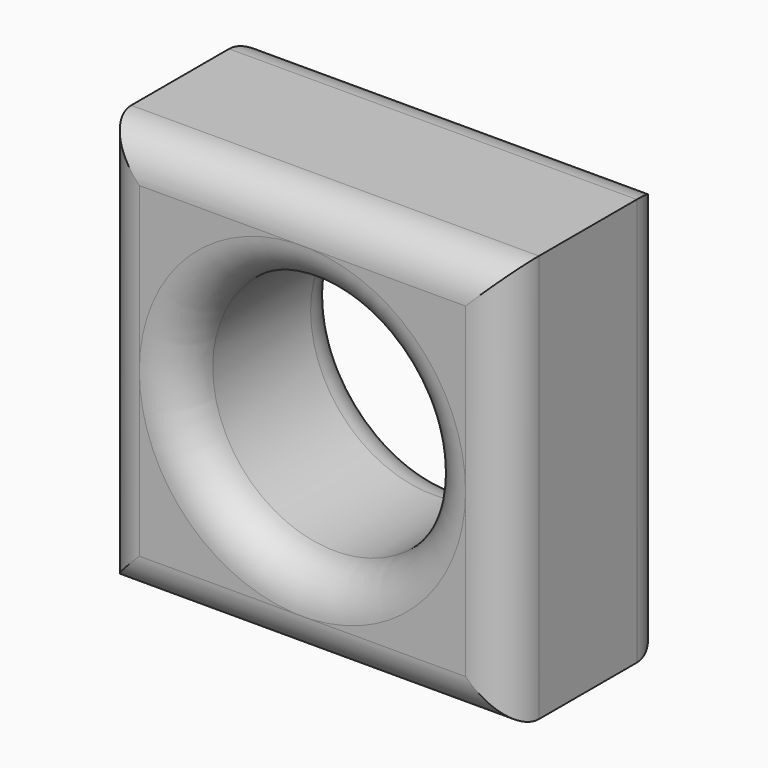
from build123d import *

# Parameters (mm, degrees)
F0_W     = 100
F0_H     = 100
F1_DEPTH = 50
F3_D     = 60
F4_R     = 9.99999


# Not quite as in the source:
# - a fillet or chamfer is up to 0.001 mm smaller than in the source, because OpenCascade refuses the exact size


with BuildPart() as f1:
    # F0 (on Front) → F1 (new body)
    with BuildSketch(Plane.XZ):
        with Locations((50, 50)):
            Rectangle(F0_W, F0_H)
    extrude(amount=F1_DEPTH)

    # F3 (through all)
    with Locations(Plane.XZ.offset(50)):
        with Locations((50, 50)):
            Hole(F3_D / 2)

    # F4 (radius 10 in the source; OpenCascade refuses exactly that, so slightly less here)
    f4_edges = [f1.edges().sort_by_distance(p)[0] for p in [
        (50, -50, 0),
        (0, -50, 50),
        (100, -50, 50),
        (50, -50, 100),
        (20, -50, 50),
        (50, 0, 0),
        (0, 0, 50),
        (100, 0, 50),
        (50, 0, 100),
        (20, 0, 50),
    ]]
    fillet(f4_edges, radius=F4_R)


solid = f1.part
